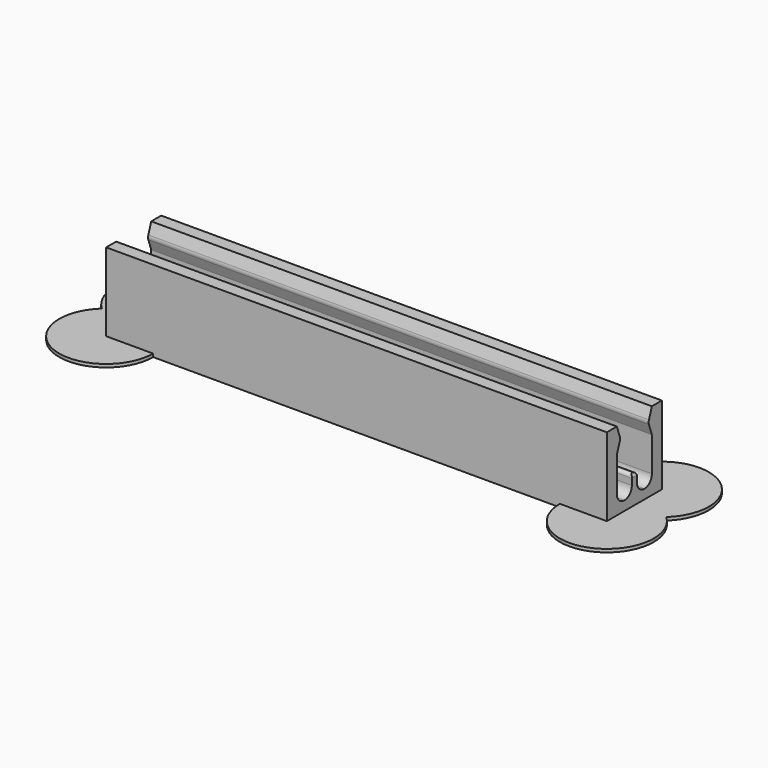
from build123d import *

# Parameters (mm, degrees)
F0_W      = 80
F0_H      = 7
F1_DEPTH  = 2
F0_H_2    = 2
F2_DEPTH  = 13
F3_W      = 1
F3_H      = 3
F4_DEPTH  = 80
F5_R      = 1
F6_R      = 1
F7_R      = 1.49999
F8_R      = 0.49999
F10_DEPTH = 0.5


# Not quite as in the source:
# - a fillet or chamfer is up to 0.001 mm smaller than in the source, because OpenCascade refuses the exact size
# - a feature names something its author has since deleted; it is built from what else it names


with BuildPart() as f1:
    # F0 (on Top) → F1 (new body)
    with BuildSketch(Plane.XY):
        Rectangle(F0_W, F0_H)
    extrude(amount=F1_DEPTH)

    # F0 (on Top) → F2 (join)
    with BuildSketch(Plane.XY):
        with Locations((0, 4.5)):
            Rectangle(F0_W, F0_H_2)
        with Locations((0, -4.5)):
            Rectangle(F0_W, F0_H_2)
    extrude(amount=F2_DEPTH)

    # F3 (on face) → F4 (join)
    with BuildSketch(Plane(origin=(-40, 0, 0), x_dir=(0, -1, 0), z_dir=(-1, 0, 0))):
        Polygon((-3.5, 13), (-3.5, 9), (-2.8, 11), align=None)
        Polygon((2.8, 11), (3.5, 9), (3.5, 13), align=None)
        with Locations((0, 3.5)):
            Rectangle(F3_W, F3_H)
    extrude(amount=-F4_DEPTH)

    # F5
    f5_edges = [f1.edges().sort_by_distance(p)[0] for p in [
        (0, 2.8, 11),
    ]]
    fillet(f5_edges, radius=F5_R)

    # F6
    f6_edges = [f1.edges().sort_by_distance(p)[0] for p in [
        (0, -2.8, 11),
    ]]
    fillet(f6_edges, radius=F6_R)

    # F7 (radius 1.5 in the source; OpenCascade refuses exactly that, so slightly less here)
    f7_edges = [f1.edges().sort_by_distance(p)[0] for p in [
        (0, -3.5, 2),
        (0, 3.5, 2),
        (0, -0.5, 2),
        (0, 0.5, 2),
    ]]
    fillet(f7_edges, radius=F7_R)

    # F8 (radius 0.5 in the source; OpenCascade refuses exactly that, so slightly less here)
    f8_edges = [f1.edges().sort_by_distance(p)[0] for p in [
        (0, -0.5, 5),
        (0, 0.5, 5),
        (-40, 0, 5),
        (40, 0, 5),
    ]]
    fillet(f8_edges, radius=F8_R)

    # F9 (on face) → F10 (join)
    with BuildSketch(Plane(origin=(0, 0, 0), x_dir=(1, 0, 0), z_dir=(0, 0, -1))):
        with BuildLine():
            ThreePointArc((-40, 2), (-42.7386127875, 1.4821200219), (-45.0990195136, 0))
            ThreePointArc((-45.0990195136, 0), (-42.7386127875, -1.4821200219), (-40, -2))
            Line((-40, -2), (-40, 2))
        make_face()
        with BuildLine():
            Line((-40, 5.5), (-32.5, 5.5))
            ThreePointArc((-32.5, 5.5), (-43.0006127414, 12.3735960876), (-45.0990195136, 0))
            ThreePointArc((-45.0990195136, 0), (-42.7386127875, 1.4821200219), (-40, 2))
            Line((-40, 2), (-40, 5.5))
        make_face()
        with BuildLine():
            ThreePointArc((-40, -2), (-42.7386127875, -1.4821200219), (-45.0990195136, 0))
            ThreePointArc((-45.0990195136, 0), (-43.0006127414, -12.3735960876), (-32.5, -5.5))
            Line((-32.5, -5.5), (-40, -5.5))
            Line((-40, -5.5), (-40, -2))
        make_face()
        with BuildLine():
            Line((40, -5.5), (32.5, -5.5))
            ThreePointArc((32.5, -5.5), (40, -13), (47.5, -5.5))
            ThreePointArc((47.5, -5.5), (46.8735960876, -2.4993872586), (45.0990195136, 0))
            ThreePointArc((45.0990195136, 0), (42.7386127875, -1.4821200219), (40, -2))
            Line((40, -2), (40, -5.5))
        make_face()
        with BuildLine():
            ThreePointArc((40, -2), (42.7386127875, -1.4821200219), (45.0990195136, 0))
            ThreePointArc((45.0990195136, 0), (42.7386127875, 1.4821200219), (40, 2))
            Line((40, 2), (40, -2))
        make_face()
        with BuildLine():
            ThreePointArc((47.5, 5.5), (40, 13), (32.5, 5.5))
            Line((32.5, 5.5), (40, 5.5))
            Line((40, 5.5), (40, 2))
            ThreePointArc((40, 2), (42.7386127875, 1.4821200219), (45.0990195136, 0))
            ThreePointArc((45.0990195136, 0), (46.8735960876, 2.4993872586), (47.5, 5.5))
        make_face()
    extrude(amount=-F10_DEPTH)


solid = f1.part
